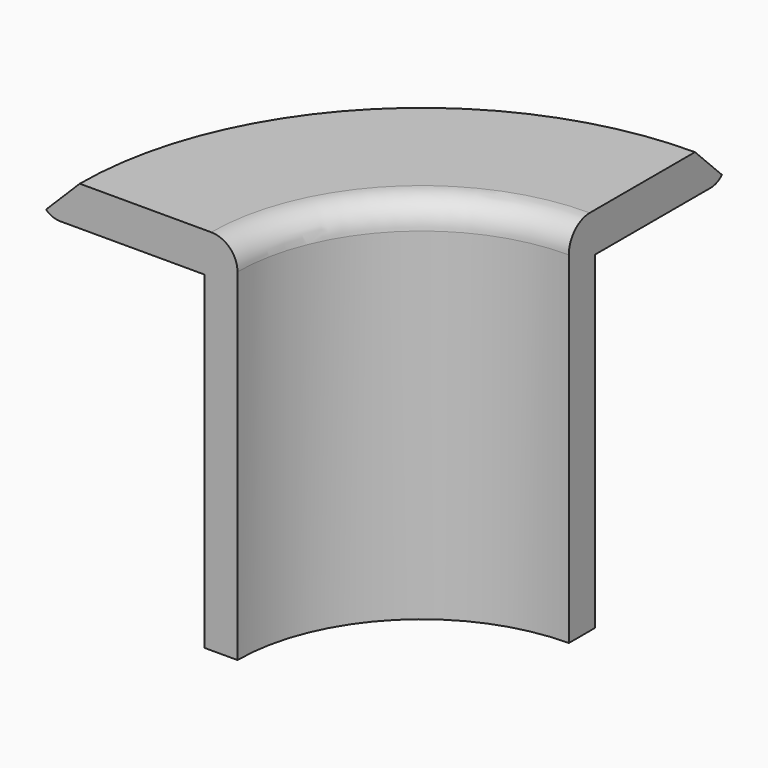
from build123d import *

# Parameters (mm, degrees)
F1_ANGLE    = 90
F2_R        = 1.5
F3_T2_ANGLE = 120.4977458854
F4_R        = 2


# Not quite as in the source:
# - a fillet or chamfer that OpenCascade refuses, or shapes differently, is made with other operations: its cross-section is extruded or revolved along the edge and cut away or added


with BuildPart() as f1:
    # F0 (on Front) → F1 (revolve)
    with BuildSketch(Plane.XZ):
        Polygon((-2.5, 0), (0, 0), (0, 28), (-15, 28), (-15, 25), (-12.5, 25), (-2.5, 25), align=None)
    revolve(axis=Axis((14, 0, -3.1492561102), (0, 0, -1)), revolution_arc=F1_ANGLE)

    # F2
    f2_edges = [f1.edges().sort_by_distance(p)[0] for p in [
        (-6.506097, 20.506097, 25),
    ]]
    fillet(f2_edges, radius=F2_R)

    # F3: chamfer of 3 on 1 edges, made by hand

    # F3_s1 → F3_t2 (revolve, cut)
    with BuildSketch(Plane(origin=(0.9684561095, -3.5525312522, 0), x_dir=(0, 0, 1), z_dir=(0.2630122362, -0.9647924977, 0))):
        Polygon((25, 15.4929050323), (28, 12.4929050323), (28, 15.4929050323), align=None)
    revolve(axis=Axis((14, 0, 28), (0, 0, -1)), revolution_arc=F3_T2_ANGLE, mode=Mode.SUBTRACT)

    # F4
    f4_edges = [f1.edges().sort_by_distance(p)[0] for p in [
        (4.100505, 9.899495, 28),
    ]]
    fillet(f4_edges, radius=F4_R)


solid = f1.part
